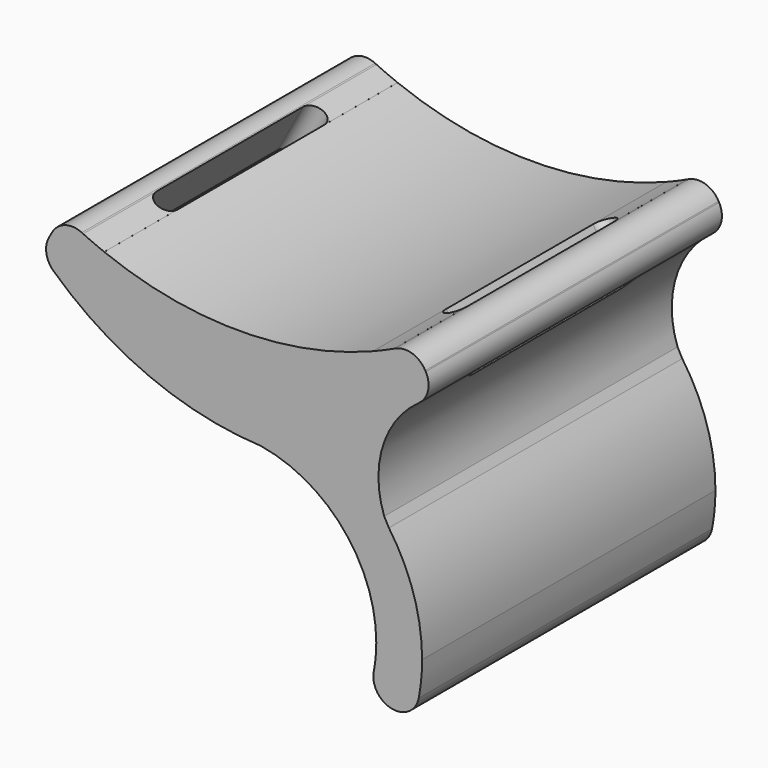
from build123d import *

# Parameters (mm, degrees)
F1_DEPTH = 50.8
F2_R     = 3.17499
F4_DEPTH = 25.4
F6_DEPTH = 25.4
F7_R     = 50.8
F8_DEPTH = 50.8
F9_R     = 3.175


# Not quite as in the source:
# - a fillet or chamfer is up to 0.001 mm smaller than in the source, because OpenCascade refuses the exact size
# - a feature names something its author has since deleted; it is built from what else it names


with BuildPart() as f1:
    # F0 (on Front) → F1 (new body)
    with BuildSketch(Plane.XZ):
        with BuildLine():
            ThreePointArc((24.0096036311, -41.4286058918), (25.0654524906, -37.313693309), (25.4207147422, -33.0803599757))
            ThreePointArc((25.4207147422, -33.0803599757), (24.2437436495, -25.4380520418), (20.821906037, -18.5039941488))
            Line((20.821906037, -18.5039941488), (20.1693195051, -17.2969153494))
            ThreePointArc((20.1693195051, -17.2969153494), (20.4643815884, -7.4727541905), (27.4307736322, -0.5394587257))
            Line((27.4307736322, -0.5394587257), (24.3787300207, 5.0289817915))
            ThreePointArc((24.3787300207, 5.0289817915), (22.9739817859, 4.2874085483), (21.5467011146, 3.5901866586))
            ThreePointArc((21.5467011146, 3.5901866586), (20.0925256969, 2.935513576), (18.6184879198, 2.3268793492))
            ThreePointArc((18.6184879198, 2.3268793492), (0, -1.2138607271), (-18.6184879198, 2.3268793492))
            ThreePointArc((-18.6184879198, 2.3268793492), (-20.0925256969, 2.935513576), (-21.5467011146, 3.5901866586))
            ThreePointArc((-21.5467011146, 3.5901866586), (-22.97860176, 4.289755995), (-24.3878181692, 5.0339641827))
            Line((-24.3878181692, 5.0339641827), (-27.4450352449, -0.5316376492))
            ThreePointArc((-27.4450352449, -0.5316376492), (-13.4987465328, -10.3152085141), (3.0701766945, -14.276017876))
            ThreePointArc((3.0701766945, -14.276017876), (14.5292424103, -20.7351129184), (19.0707147422, -33.0803599757))
            ThreePointArc((19.0707147422, -33.0803599757), (18.8042680535, -36.2553599757), (18.0123814088, -39.3415444128))
            Line((18.0123814088, -39.3415444128), (24.0096036311, -41.4286058918))
        make_face()
        with BuildLine():
            ThreePointArc((18.6184879198, 2.3268793492), (20.0925256969, 2.935513576), (21.5467011146, 3.5901866586))
            Line((21.5467011146, 3.5901866586), (19.869957668, 6.6493979065))
            Line((19.869957668, 6.6493979065), (17.0857374094, 5.1233761008))
            Line((17.0857374094, 5.1233761008), (18.6184879198, 2.3268793492))
        make_face()
        with BuildLine():
            ThreePointArc((-21.5467011146, 3.5901866586), (-20.0925256969, 2.935513576), (-18.6184879198, 2.3268793492))
            Line((-18.6184879198, 2.3268793492), (-17.0857374094, 5.1233761008))
            Line((-17.0857374094, 5.1233761008), (-19.869957668, 6.6493979065))
            Line((-19.869957668, 6.6493979065), (-21.5467011146, 3.5901866586))
        make_face()
    extrude(amount=F1_DEPTH)

    # F2 (radius 3.175 in the source; OpenCascade refuses exactly that, so slightly less here)
    f2_edges = [f1.edges().sort_by_distance(p)[0] for p in [
        (24.009604, -25.4, -41.428606),
        (18.012381, -25.4, -39.341544),
    ]]
    fillet(f2_edges, radius=F2_R)

    # F3 (on face) → F4 (cut)
    with BuildSketch(Plane(origin=(1.7876055886, 0, -3.2614787517), x_dir=(0.8769197665, 0, 0.4806367892), z_dir=(-0.4806367892, 0, 0.8769197665))):
        with BuildLine():
            Line((20.6203038983, -38.1), (20.6203038983, -12.7))
            ThreePointArc((20.6203038983, -12.7), (19.0328038983, -11.1125), (17.4453038983, -12.7))
            Line((17.4453038983, -12.7), (17.4453038983, -38.1))
            ThreePointArc((17.4453038983, -38.1), (19.0328038983, -39.6875), (20.6203038983, -38.1))
        make_face()
    extrude(amount=-F4_DEPTH, mode=Mode.SUBTRACT)

    # F5 (on face) → F6 (cut)
    with BuildSketch(Plane(origin=(-1.7876055886, 0, -3.2614787517), x_dir=(0.8769197665, 0, -0.4806367892), z_dir=(0.4806367892, 0, 0.8769197665))):
        with BuildLine():
            ThreePointArc((-20.6203038983, -38.1), (-19.0328038983, -39.6875), (-17.4453038983, -38.1))
            Line((-17.4453038983, -38.1), (-17.4453038983, -12.7))
            ThreePointArc((-17.4453038983, -12.7), (-19.0328038983, -11.1125), (-20.6203038983, -12.7))
            Line((-20.6203038983, -12.7), (-20.6203038983, -38.1))
        make_face()
    extrude(amount=-F6_DEPTH, mode=Mode.SUBTRACT)

    # F7 (on face) → F8 (cut)
    with BuildSketch(Plane(origin=(0, 0, 0), x_dir=(-1, 0, 0), z_dir=(0, 1, 0))):
        with Locations((-9.1173e-06, 49.5971090476)):
            Circle(F7_R)
    extrude(amount=-F8_DEPTH, mode=Mode.SUBTRACT)

    # F9
    f9_edges = [f1.edges().sort_by_distance(p)[0] for p in [
        (24.37873, -25.4, 5.028982),
        (27.430774, -25.4, -0.539459),
        (-24.387818, -25.4, 5.033964),
        (-27.445035, -25.4, -0.531638),
    ]]
    fillet(f9_edges, radius=F9_R)


solid = f1.part
